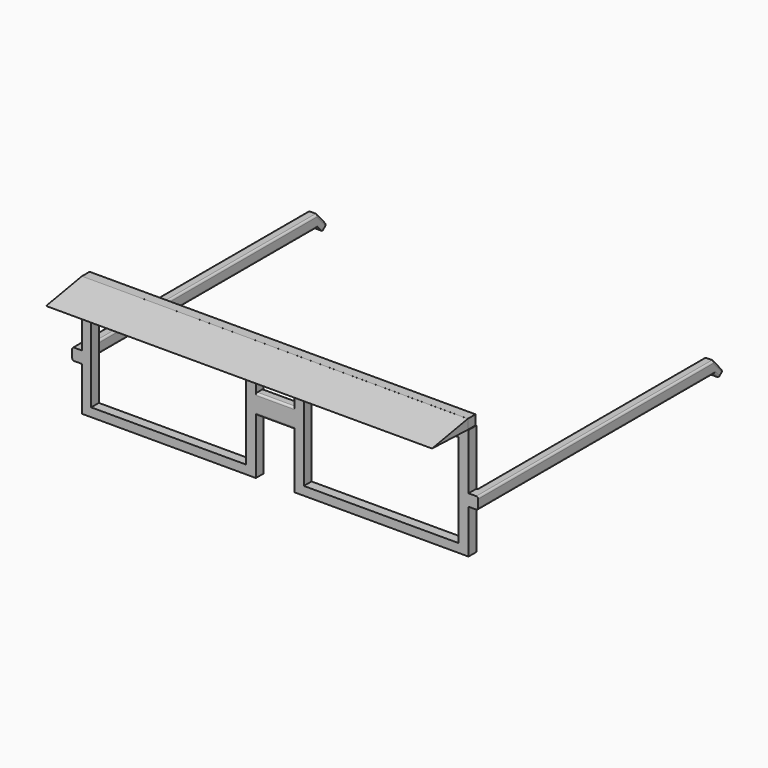
from build123d import *

# Parameters (mm, degrees)
F0_W     = 26.4591541143
F0_H     = 51.1078872686
F0_W_2   = 101.6
F0_W_3   = 24.3408458857
F0_H_2   = 24.597927928
F1_DEPTH = 25.4
F2_W     = 25.4
F2_H     = 31.037738815
F3_DEPTH = 25.4
F4_W     = 25.4
F4_H     = 31.0394611481
F5_DEPTH = 25.4
F7_DEPTH = 25.4
F9_DEPTH = 1014.095
F10_R    = 5.08
F11_R    = 5.08


# Not quite as in the source:
# - two fillets or chamfers of one size are made in one step


with BuildPart() as f1:
    # F0 (on Front) → F1 (new body)
    with BuildSketch(Plane.XZ):
        Polygon((-730.28846806, 0), (-730.28846806, 245.0714976708), (-323.88846806, 245.0714976708), (-323.88846806, 173.643636104), (-297.4293139458, 173.643636104), (-297.4293139458, 210.000038147), (-297.4293139458, 234.5979660749), (-297.4293139458, 270.0304389), (-754.6293139458, 270.0304389), (-754.6293139458, -22.7653142065), (-297.4293139458, -22.7653142065), (-297.4293139458, 122.5357488354), (-323.88846806, 122.5357488354), (-323.88846806, 0), align=None)
        with Locations((-310.6588910029, 148.0896924697)):
            Rectangle(F0_W, F0_H)
        with Locations((-246.6293139458, 148.0896924697)):
            Rectangle(F0_W_2, F0_H)
        Polygon((-195.8293139458, 210.000038147), (-195.8293139458, 173.643636104), (-171.48846806, 173.643636104), (-171.48846806, 245.0714976708), (234.91153194, 245.0714976708), (234.91153194, 0), (-171.48846806, 0), (-171.48846806, 122.5357488354), (-195.8293139458, 122.5357488354), (-195.8293139458, -22.7653142065), (261.3706860542, -22.7653142065), (261.3706860542, 270.0304389), (-195.8293139458, 270.0304389), (-195.8293139458, 234.5979660749), align=None)
        with Locations((-183.6588910029, 148.0896924697)):
            Rectangle(F0_W_3, F0_H)
        with Locations((-246.6293139458, 222.299002111)):
            Rectangle(F0_W_2, F0_H_2)
    extrude(amount=F1_DEPTH)

    # F2 (on face) → F3 (join)
    with BuildSketch(Plane(origin=(-754.6293139458, 0, 0), x_dir=(0, -1, 0), z_dir=(-1, 0, 0))):
        Polygon((0, 92.5948235318), (0, 123.6325623468), (-749.2181062698, 123.6325623468), (-778.2575488091, 90.4286950827), (-763.7378275394, 77.7300353711), (-750.7373791816, 92.5948235318), align=None)
        with Locations((12.7, 108.1136929393)):
            Rectangle(F2_W, F2_H)
    extrude(amount=F3_DEPTH)

    # F4 (on face) → F5 (join)
    with BuildSketch(Plane.YZ.offset(261.3706860542)):
        with Locations((-12.7, 108.1128317727)):
            Rectangle(F4_W, F4_H)
        Polygon((749.224126339, 123.6325623468), (0, 123.6325623468), (0, 92.5931011987), (750.7367628879, 92.5931011987), (763.7009845333, 77.7766145807), (778.2266139984, 90.4863402247), align=None)
    extrude(amount=F5_DEPTH)

    # F6 (on face) → F7 (join)
    with BuildSketch(Plane.XY.offset(270.0304389)):
        Polygon((259.4215273857, 0), (-754.6293139458, 0), (-754.6293139458, -25.4), (259.4215273857, -25.2286773175), align=None)
    extrude(amount=F7_DEPTH)

    # F10
    f10_edges = [f1.edges().sort_by_distance(p)[0] for p in [
        (-246.629314, -25.4, 173.643636),
        (-246.629314, -25.4, 122.535749),
        (-246.629314, 0, 173.643636),
        (-246.629314, 0, 122.535749),
    ]]
    fillet(f10_edges, radius=F10_R)

    # F11
    f11_edges = [f1.edges().sort_by_distance(p)[0] for p in [
        (-754.629314, 374.609053, 123.632562),
        (-780.029314, 361.909053, 123.632562),
        (-780.029314, 362.66869, 92.594824),
        (-754.629314, 375.36869, 92.594824),
        (-767.329314, 778.257549, 90.428695),
        (-780.029314, 763.737828, 107.030629),
        (-767.329314, 763.737828, 77.730035),
        (-754.629314, 763.737828, 107.030629),
        (261.370686, 375.368381, 92.593101),
        (286.770686, 362.668381, 92.593101),
        (286.770686, 757.218874, 85.184858),
        (286.770686, 763.72537, 107.059451),
        (286.770686, 361.912063, 123.632562),
        (261.370686, 374.612063, 123.632562),
        (274.070686, 763.700985, 77.776615),
        (261.370686, 763.72537, 107.059451),
        (261.370686, 770.963799, 84.131477),
        (274.070686, 778.226614, 90.48634),
    ]]
    fillet(f11_edges, radius=F11_R)


with BuildPart() as f9:
    # F8 (on face) → F9 (new body)
    with BuildSketch(Plane(origin=(-754.6293139458, 0, 0), x_dir=(0, -1, 0), z_dir=(-1, 0, 0))):
        Polygon((142.9468989372, 274.3944525719), (25.4, 295.4304389), (25.4, 270.0304389), align=None)
    extrude(amount=-F9_DEPTH)


solid = Compound([f1.part, f9.part])
